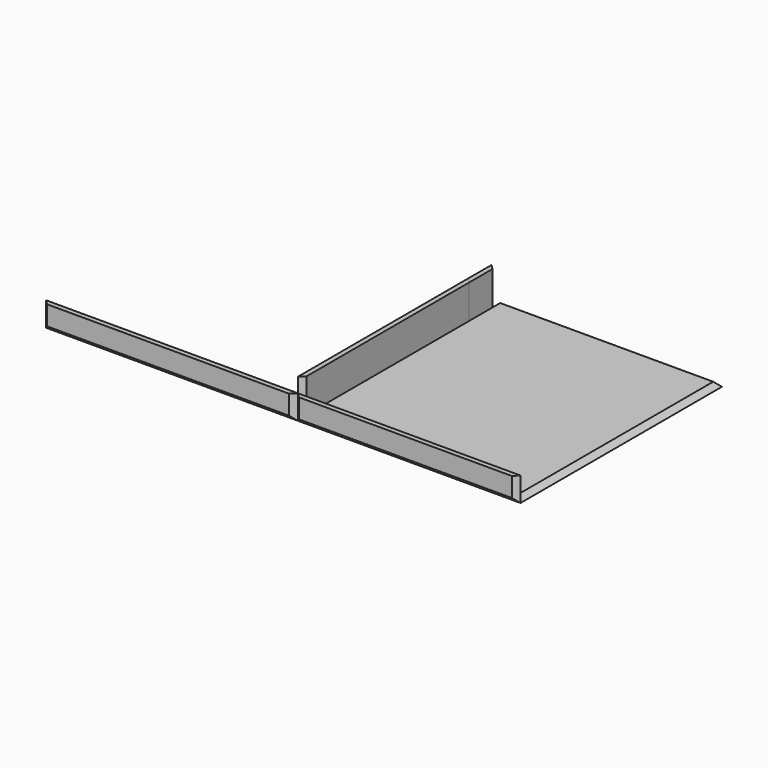
from build123d import *

# Parameters (mm, degrees)
F0_W      = 92
F0_H      = 104
F1_DEPTH  = 2
F2_SIZE   = 1.99999
F3_W      = 104
F3_H      = 10
F4_DEPTH  = 2
F5_SIZE   = 1.99999
F6_W      = 92
F6_H      = 10
F7_DEPTH  = 2
F8_SIZE   = 1.99999
F9_W      = 100
F9_H      = 16
F10_DEPTH = 2
F11_SIZE  = 1.99999
F12_W     = 88
F12_H     = 16
F13_DEPTH = 2
F14_SIZE  = 1.99999


# Not quite as in the source:
# - a fillet or chamfer is up to 0.001 mm smaller than in the source, because OpenCascade refuses the exact size


with BuildPart() as f1:
    # F0 (on Top) → F1 (new body)
    with BuildSketch(Plane.XY):
        with Locations((46, 52)):
            Rectangle(F0_W, F0_H)
    extrude(amount=F1_DEPTH)

    # F2 (size 2 in the source; OpenCascade refuses exactly that, so slightly less here)
    f2_edges = [f1.edges().sort_by_distance(p)[0] for p in [
        (0, 52, 2),
        (46, 0, 2),
        (92, 52, 2),
        (46, 104, 2),
    ]]
    chamfer(f2_edges, length=F2_SIZE)


with BuildPart() as f4:
    # F3 (on Front) → F4 (new body)
    with BuildSketch(Plane.XZ):
        with Locations((-52, 5)):
            Rectangle(F3_W, F3_H)
    extrude(amount=F4_DEPTH)

    # F5 (size 2 in the source; OpenCascade refuses exactly that, so slightly less here)
    f5_edges = [f4.edges().sort_by_distance(p)[0] for p in [
        (-52, -2, 0),
        (0, -2, 5),
        (-104, -2, 5),
    ]]
    chamfer(f5_edges, length=F5_SIZE)


with BuildPart() as f7:
    # F6 (on Front) → F7 (new body)
    with BuildSketch(Plane.XZ):
        with Locations((46, 5)):
            Rectangle(F6_W, F6_H)
    extrude(amount=F7_DEPTH)

    # F8 (size 2 in the source; OpenCascade refuses exactly that, so slightly less here)
    f8_edges = [f7.edges().sort_by_distance(p)[0] for p in [
        (0, -2, 5),
        (46, -2, 0),
        (92, -2, 5),
    ]]
    chamfer(f8_edges, length=F8_SIZE)


with BuildPart() as f10:
    # F9 (on Right) → F10 (new body)
    with BuildSketch(Plane.YZ):
        with Locations((50, 8)):
            Rectangle(F9_W, F9_H)
    extrude(amount=F10_DEPTH)

    # F11 (size 2 in the source; OpenCascade refuses exactly that, so slightly less here)
    f11_edges = [f10.edges().sort_by_distance(p)[0] for p in [
        (2, 100, 8),
        (2, 0, 8),
    ]]
    chamfer(f11_edges, length=F11_SIZE)


with BuildPart() as f13:
    # F12 (on Right) → F13 (new body)
    with BuildSketch(Plane.YZ):
        with Locations((44, 8)):
            Rectangle(F12_W, F12_H)
    extrude(amount=F13_DEPTH)

    # F14 (size 2 in the source; OpenCascade refuses exactly that, so slightly less here)
    f14_edges = [f13.edges().sort_by_distance(p)[0] for p in [
        (2, 0, 8),
        (2, 88, 8),
    ]]
    chamfer(f14_edges, length=F14_SIZE)


solid = Compound([f1.part, f4.part, f7.part, f10.part, f13.part])
